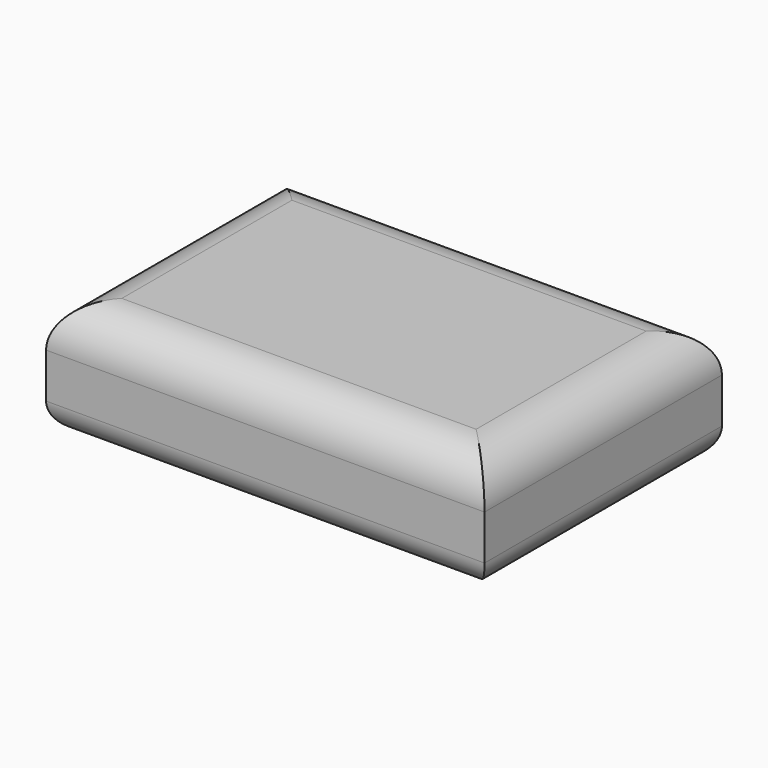
from build123d import *

# Parameters (mm, degrees)
F0_W        = 74.2
F0_H        = 48.8
F1_DEPTH    = 2.54
F2_W        = 79.4061459601
F2_H        = 53.7425726652
F2_W_2      = 74.2
F2_H_2      = 48.8
F3_DEPTH    = 20.828
F4_R        = 7.62
F5_T1_DEPTH = 79.1425726652
F5_T3_DEPTH = 104.8061459601


# Not quite as in the source:
# - a fillet or chamfer that OpenCascade refuses, or shapes differently, is made with other operations: its cross-section is extruded or revolved along the edge and cut away or added


with BuildPart() as f1:
    # F0 (on Top) → F1 (new body)
    with BuildSketch(Plane.XY):
        with Locations((0.8302908391, 2.9207762395)):
            Rectangle(F0_W, F0_H)
    extrude(amount=F1_DEPTH)

    # F2 (on face) → F3 (join)
    with BuildSketch(Plane.XY.offset(2.54)):
        with Locations((1.1322144419, 3.0947271734)):
            Rectangle(F2_W, F2_H)
        with Locations((0.8302908391, 2.9207762395)):
            Rectangle(F2_W_2, F2_H_2, mode=Mode.SUBTRACT)
    extrude(amount=-F3_DEPTH)

    # F4
    f4_edges = [f1.edges().sort_by_distance(p)[0] for p in [
        (1.132214, 29.966014, 2.54),
        (-38.570859, 3.094727, 2.54),
        (40.835287, 3.094727, 2.54),
        (1.132214, -23.776559, 2.54),
    ]]
    fillet(f4_edges, radius=F4_R)

    # F5: fillet of radius 5.08 on 4 edges, made by hand

    # F5_s2 → F5_t1 (cut)
    with BuildSketch(Plane.XZ.offset(-42.6660135061)):
        with BuildLine():
            ThreePointArc((40.8352874219, -13.208), (39.3473898704, -16.8001024484), (35.7552874219, -18.288))
            Line((35.7552874219, -18.288), (40.8352874219, -18.288))
            Line((40.8352874219, -18.288), (40.8352874219, -13.208))
        make_face()
        with BuildLine():
            ThreePointArc((-33.4908585382, -18.288), (-37.0829609866, -16.8001024484), (-38.5708585382, -13.208))
            Line((-38.5708585382, -13.208), (-38.5708585382, -18.288))
            Line((-38.5708585382, -18.288), (-33.4908585382, -18.288))
        make_face()
    extrude(amount=F5_T1_DEPTH, mode=Mode.SUBTRACT)

    # F5_s4 → F5_t3 (cut)
    with BuildSketch(Plane.YZ.offset(-51.2708585382)):
        with BuildLine():
            ThreePointArc((-18.6965591592, -18.288), (-22.2886616076, -16.8001024484), (-23.7765591592, -13.208))
            Line((-23.7765591592, -13.208), (-23.7765591592, -18.288))
            Line((-23.7765591592, -18.288), (-18.6965591592, -18.288))
        make_face()
        with BuildLine():
            ThreePointArc((29.9660135061, -13.208), (28.4781159545, -16.8001024484), (24.8860135061, -18.288))
            Line((24.8860135061, -18.288), (29.9660135061, -18.288))
            Line((29.9660135061, -18.288), (29.9660135061, -13.208))
        make_face()
    extrude(amount=F5_T3_DEPTH, mode=Mode.SUBTRACT)


solid = f1.part
